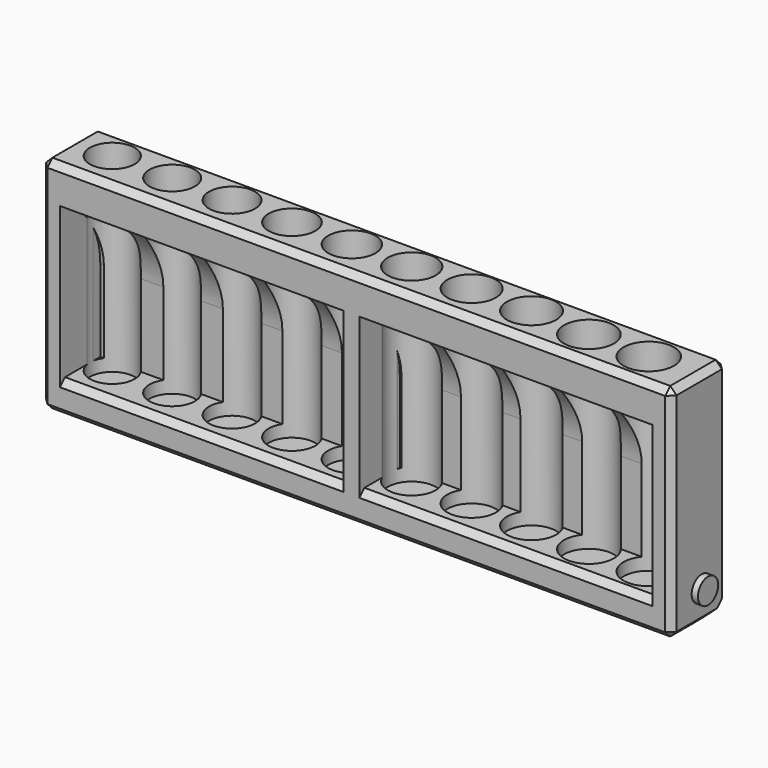
from build123d import *

# Parameters (mm, degrees)
F0_W          = 100
F0_H          = 11
F2_DEPTH      = 35
F3_START      = 3
F1_R          = 4
F1_R_2        = 3.95
F1_R_3        = 3.9
F1_R_4        = 3.85
F1_R_5        = 3.8
F1_R_6        = 3.75
F1_R_7        = 3.7
F1_R_8        = 3.65
F1_R_9        = 3.6
F1_R_10       = 3.55
F3_DEPTH      = 37
F5_START      = -3
F5_DEPTH      = 46.5
F6_START      = -52
F6_DEPTH      = 45
F7_SIZE       = 1
F8_R          = 2
F9_DEPTH      = 2
F9_DEPTH_BACK = 1
F10_START     = -99
F10_DEPTH     = 2
F11_T1_DEPTH  = 123


# Not quite as in the source:
# - a fillet or chamfer that OpenCascade refuses, or shapes differently, is made with other operations: its cross-section is extruded or revolved along the edge and cut away or added


with BuildPart() as f2:
    # F0 (on Top) → F2 (new body)
    with BuildSketch(Plane.XY):
        with Locations((-50, -5.5)):
            Rectangle(F0_W, F0_H)
    extrude(amount=F2_DEPTH)

    # F1 (on Top) → F3 (cut)
    with BuildSketch(Plane.XY.offset(F3_START)):
        with Locations((-8, -5.5)):
            Circle(F1_R)
        with Locations((-17.5, -5.5)):
            Circle(F1_R_2)
        with Locations((-27, -5)):
            Circle(F1_R_3)
        with Locations((-36.5, -5)):
            Circle(F1_R_4)
        with Locations((-46, -5)):
            Circle(F1_R_5)
        with Locations((-55.5, -5)):
            Circle(F1_R_6)
        with Locations((-65, -5)):
            Circle(F1_R_7)
        with Locations((-74.5, -5)):
            Circle(F1_R_8)
        with Locations((-84, -5)):
            Circle(F1_R_9)
        with Locations((-93.5, -5)):
            Circle(F1_R_10)
    extrude(amount=F3_DEPTH, mode=Mode.SUBTRACT)

    # F4 (on Right) → F5 (cut)
    with BuildSketch(Plane.YZ.offset(F5_START)):
        with BuildLine():
            Line((-13, 29.8321595662), (-13, 5))
            Line((-13, 5), (-3, 5))
            Line((-3, 5), (-3, 18))
            ThreePointArc((-3, 18), (-5.8348486101, 25.7459666924), (-13, 29.8321595662))
        make_face()
        with BuildLine():
            ThreePointArc((-15, 30), (-13.9964848766, 29.9579662735), (-13, 29.8321595662))
            Line((-13, 29.8321595662), (-13, 30))
            Line((-13, 30), (-15, 30))
        make_face()
    extrude(amount=-F5_DEPTH, mode=Mode.SUBTRACT)

    # F4 (on Right) → F6 (cut)
    with BuildSketch(Plane.YZ.offset(F6_START)):
        with BuildLine():
            Line((-13, 29.8321595662), (-13, 5))
            Line((-13, 5), (-3, 5))
            Line((-3, 5), (-3, 18))
            ThreePointArc((-3, 18), (-5.8348486101, 25.7459666924), (-13, 29.8321595662))
        make_face()
        with BuildLine():
            ThreePointArc((-15, 30), (-13.9964848766, 29.9579662735), (-13, 29.8321595662))
            Line((-13, 29.8321595662), (-13, 30))
            Line((-13, 30), (-15, 30))
        make_face()
    extrude(amount=-F6_DEPTH, mode=Mode.SUBTRACT)

    # F7
    f7_edges = [f2.edges().sort_by_distance(p)[0] for p in [
        (-50, -11, 35),
        (-100, -5.5, 35),
        (-50, 0, 35),
        (0, -5.5, 35),
        (0, -11, 17.5),
        (0, 0, 17.5),
        (0, -5.5, 0),
        (-50, -11, 0),
        (-100, -11, 17.5),
        (-74.5, -11, 5),
        (-26.25, -11, 5),
        (-100, -5.5, 0),
        (-100, 0, 17.5),
    ]]
    chamfer(f7_edges, length=F7_SIZE)

    # F8 (on Right) → F9 (join, two sides)
    with BuildSketch(Plane.YZ) as f9_sk:
        with Locations((-5, 5)):
            Circle(F8_R)
    extrude(amount=-F9_DEPTH)
    extrude(f9_sk.sketch, amount=F9_DEPTH_BACK)

    # F8 (on Right) → F10 (join)
    with BuildSketch(Plane.YZ.offset(F10_START)):
        with Locations((-5, 5)):
            Circle(F8_R)
    extrude(amount=-F10_DEPTH)

    # F11: fillet of radius 5 on 1 edges, made by hand

    # F11_s2 → F11_t1 (cut)
    with BuildSketch(Plane.YZ.offset(-111.5)):
        with BuildLine():
            ThreePointArc((0, 5), (-1.4644660941, 1.4644660941), (-5, 0))
            Line((-5, 0), (0, 0))
            Line((0, 0), (0, 5))
        make_face()
    extrude(amount=F11_T1_DEPTH, mode=Mode.SUBTRACT)


solid = f2.part
